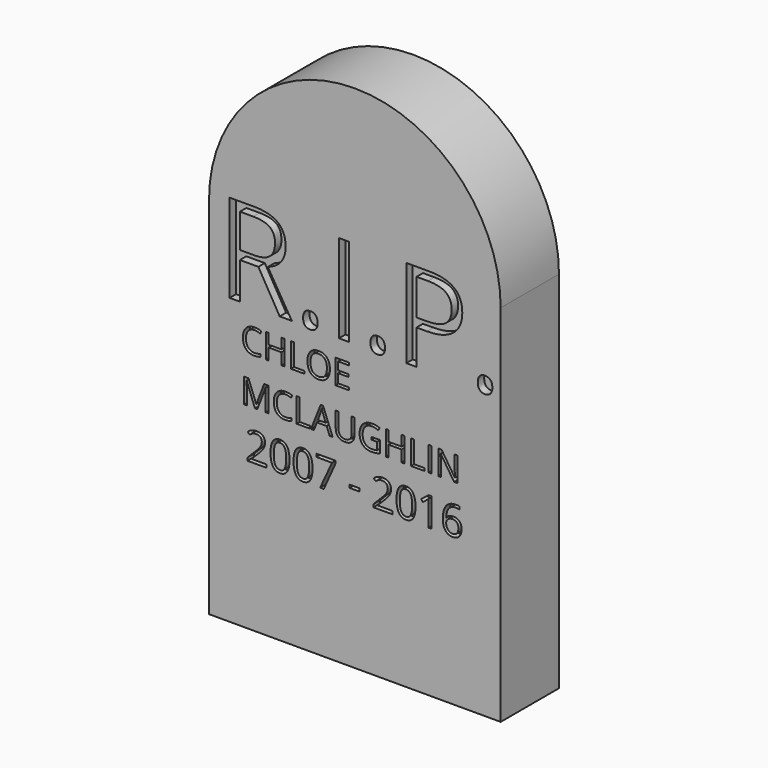
from build123d import *

# Parameters (mm, degrees)
F1_DEPTH     = 25.4
F2_TEXT_SIZE = 43.0632479093
F3_DEPTH     = 2.794
F4_TEXT_SIZE = 11.9103209105
F5_DEPTH     = 2.794
F6_TEXT_SIZE = 14.0299194476
F7_DEPTH     = 2.794


# Not quite as in the source:
# - Text() gives the source's letters only with a copy of the font that has no kerning and outlines rounded to 1/6400 em; it was checked with that copy


with BuildPart() as f1:
    # F0 (on Front) → F1 (new body)
    with BuildSketch(Plane.XZ):
        with BuildLine():
            Line((0, 127), (0, 0))
            Line((0, 0), (101.6, 0))
            Line((101.6, 0), (101.6, 127))
            ThreePointArc((101.6, 127), (50.8, 177.8), (0, 127))
        make_face()
    extrude(amount=F1_DEPTH)

    # F2 (on face) → F3 (cut)
    with BuildSketch(Plane.XZ.offset(25.4)):
        with Locations((2.9689272579, 99.3423100389)):
            Text('R.I.P.', F2_TEXT_SIZE, font='Open Sans', text_align=(TextAlign.LEFT, TextAlign.BOTTOM))
    extrude(amount=-F3_DEPTH, mode=Mode.SUBTRACT)

    # F4 (on face) → F5 (cut, through all)
    with BuildSketch(Plane.XZ.offset(25.4)):
        with Locations((11.0831256457, 84.5253486055)):
            Text('CHLOE', F4_TEXT_SIZE, font='Open Sans', text_align=(TextAlign.LEFT, TextAlign.BOTTOM))
        with Locations((11.0831256457, 68.3273121672)):
            Text('MCLAUGHLIN', F4_TEXT_SIZE, font='Open Sans', text_align=(TextAlign.LEFT, TextAlign.BOTTOM))
    extrude(amount=-F5_DEPTH, mode=Mode.SUBTRACT)

    # F6 (on face) → F7 (cut, through all)
    with BuildSketch(Plane.XZ.offset(25.4)):
        with Locations((12.7, 51.3990153984)):
            Text('2007 - 2016', F6_TEXT_SIZE, font='Open Sans', text_align=(TextAlign.LEFT, TextAlign.BOTTOM))
    extrude(amount=-F7_DEPTH, mode=Mode.SUBTRACT)


solid = f1.part
